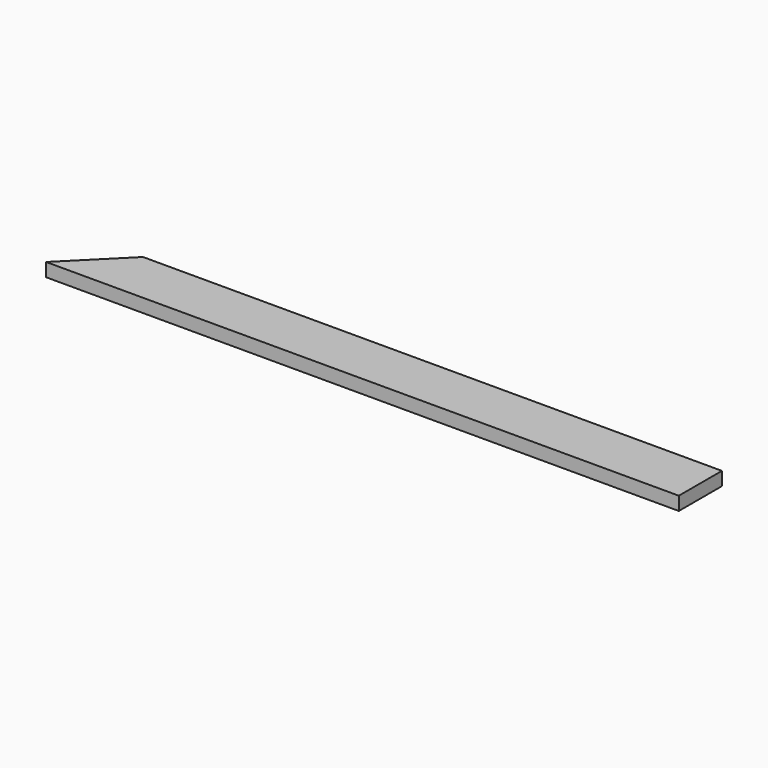
from build123d import *

# Parameters (mm, degrees)
F0_W     = 423
F0_H     = 36
F1_DEPTH = 9
F2_SIZE  = 35.99999


# Not quite as in the source:
# - a fillet or chamfer is up to 0.001 mm smaller than in the source, because OpenCascade refuses the exact size


with BuildPart() as f1:
    # F0 (on Top) → F1 (new body)
    with BuildSketch(Plane.XY):
        Rectangle(F0_W, F0_H)
    extrude(amount=F1_DEPTH)

    # F2 (size 36 in the source; OpenCascade refuses exactly that, so slightly less here)
    f2_edges = [f1.edges().sort_by_distance(p)[0] for p in [
        (-211.5, 18, 4.5),
    ]]
    chamfer(f2_edges, length=F2_SIZE)


solid = f1.part
